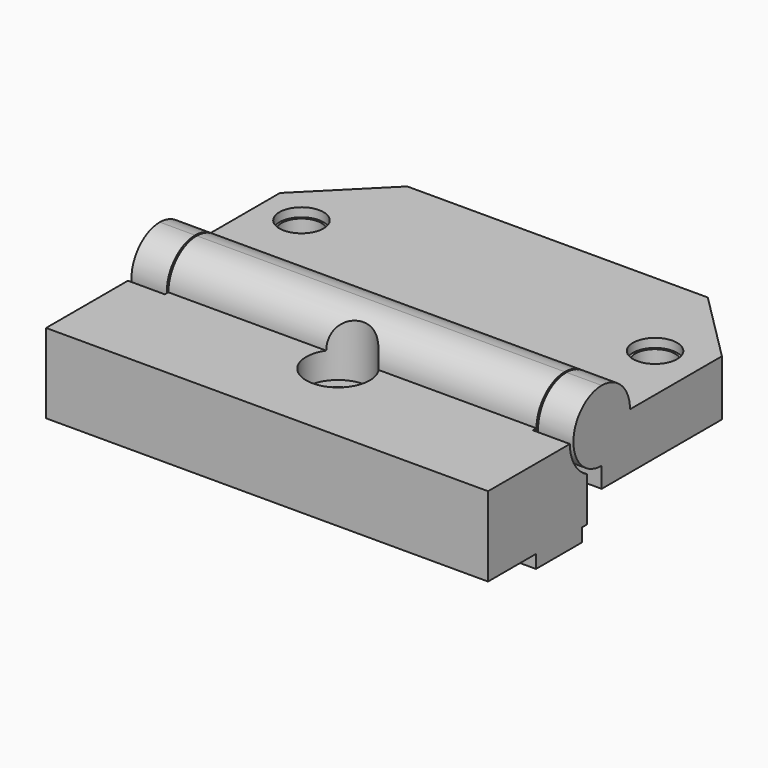
from build123d import *

# Parameters (mm, degrees)
F4_W           = 41.6464466094
F4_H           = 8
F6_W           = 4
F6_H           = 8
F7_DEPTH       = 25
F8_DEPTH       = 42
F10_DEPTH      = 46.001
F14_DEPTH      = 4
F14_DEPTH_BACK = 46
F15_DEPTH      = 41.6464466094
F16_DEPTH      = 4.1767766953
F16_DEPTH_BACK = 45.8232233047
F17_W          = 49.9999999998
F17_H          = 8.9284215122
F17_R          = 2.25
F18_DEPTH      = 25
F20_DEPTH      = 5
F21_R          = 2.25
F22_DEPTH      = 25
F23_R          = 3.6
F24_DEPTH      = 3
F24_DEPTH_BACK = 25
F25_W          = 50.0000000003
F25_H          = 6.5
F25_R          = 2.25
F26_DEPTH      = 1.5
F27_R          = 2.25
F28_DEPTH      = 25
F30_DEPTH      = 2.3
F31_R          = 2.25
F32_DEPTH      = 25
F33_SIZE       = 8
F34_R          = 2
F35_DEPTH      = 4.2
F36_R          = 2.5
F37_DEPTH      = 1


with BuildPart() as f1:
    # F0 (on Top) → F1 (revolve)
    with BuildSketch(Plane.XY):
        Polygon((-25, 0), (-17, 0), (-21, 4), (-25, 4), align=None)
    revolve(axis=Axis((-8.4116116524, 0, 0), (-1, 0, 0)))

    # F6 (on offset) → F7, piece 2 (join, through all)
    with BuildSketch(Plane.XZ.offset(-25)):
        with Locations((-23, 0)):
            Rectangle(F6_W, F6_H)
    extrude(amount=F7_DEPTH)


with BuildPart() as f1b:
    # F0 (on Top) → F1, piece 2 (revolve)
    with BuildSketch(Plane.XY):
        Polygon((-16.8232233047, 0), (0, 0), (0, 4), (-20.8232233047, 4), align=None)
        Polygon((0, 4), (0, 0), (16.8232233047, 0), (20.8232233047, 4), align=None)
    revolve(axis=Axis((-8.4116116524, 0, 0), (-1, 0, 0)))

    # F4 (on offset) → F5 (join, up to the next surface of F1b)
    with BuildSketch(Plane.XZ.offset(25)):
        Rectangle(F4_W, F4_H)
    extrude(until=Until.NEXT, dir=(0, 1, 0))

    # F13 (on face) → F15 (cut, through all)
    with BuildSketch(Plane.YZ.offset(20.8232233047)):
        with BuildLine():
            Line((-25, 4), (-25, 0))
            Line((-25, 0), (-4.5, 0))
            Line((-4.5, 0), (-4, 0))
            ThreePointArc((-4, 0), (-2.8284271247, 2.8284271247), (0, 4))
            Line((0, 4), (-25, 4))
        make_face()
    extrude(amount=-F15_DEPTH, mode=Mode.SUBTRACT)

    # F13 (on face) → F16 (join, two sides)
    with BuildSketch(Plane.YZ.offset(20.8232233047)) as f16_sk:
        with BuildLine():
            Line((-4.5, 0), (-25, 0))
            Line((-25, 0), (-25, -4))
            Line((-25, -4), (-2.0615528128, -4))
            ThreePointArc((-2.0615528128, -4), (-3.8423292192, -2.3423292192), (-4.5, 0))
        make_face()
    extrude(amount=F16_DEPTH)
    extrude(f16_sk.sketch, amount=-F16_DEPTH_BACK)

    # F17 (on face) → F18 (cut)
    with BuildSketch(Plane.XY):
        with Locations((-1e-10, -20.5357892439)):
            Rectangle(F17_W, F17_H)
        with Locations((-1e-10, -6.0417063069)):
            Circle(F17_R)
    extrude(amount=-F18_DEPTH, mode=Mode.SUBTRACT)

    # F19 (on face) → F20 (join)
    with BuildSketch(Plane(origin=(0, 0, -4), x_dir=(1, 0, 0), z_dir=(0, 0, -1))):
        Polygon((25, 16.0715784878), (-25, 16.0715784878), (-25, 2.0615528128), (-20.8232233047, 2.0615528128), (-20.8232233047, 0), (20.8232233047, 0), (20.8232233047, 2.0615528128), (25, 2.0615528128), align=None)
    extrude(amount=F20_DEPTH)

    # F21 (on face) → F22 (cut)
    with BuildSketch(Plane.XY):
        with Locations((-1e-10, -6.0417063069)):
            Circle(F21_R)
    extrude(amount=-F22_DEPTH, mode=Mode.SUBTRACT)

    # F23 (on face) → F24 (cut, two sides)
    with BuildSketch(Plane.XY) as f24_sk:
        with Locations((-1e-10, -6.0417063069)):
            Circle(F23_R)
    extrude(amount=-F24_DEPTH, mode=Mode.SUBTRACT)
    extrude(f24_sk.sketch, amount=F24_DEPTH_BACK, mode=Mode.SUBTRACT)

    # F25 (on face) → F26 (join)
    with BuildSketch(Plane(origin=(0, 0, -9), x_dir=(1, 0, 0), z_dir=(0, 0, -1))):
        with Locations((-1e-10, 6.0417063069)):
            Rectangle(F25_W, F25_H)
        with Locations((-1e-10, 6.0417063069)):
            Circle(F25_R, mode=Mode.SUBTRACT)
    extrude(amount=F26_DEPTH)


with BuildPart() as f1c:
    # F0 (on Top) → F1, piece 3 (revolve)
    with BuildSketch(Plane.XY):
        Polygon((25, 4), (21, 4), (17, 0), (25, 0), align=None)
    revolve(axis=Axis((-8.4116116524, 0, 0), (-1, 0, 0)))

    # F6 (on offset) → F7 (join, through all)
    with BuildSketch(Plane.XZ.offset(-25)):
        with Locations((23, 0)):
            Rectangle(F6_W, F6_H)
    extrude(amount=F7_DEPTH)


with BuildPart() as f8:
    # F8 (new, through all): a face of the model
    f8_faces = [f1.part.faces().sort_by_distance(p)[0] for p in [
        (-21, 14.0525639311, 0),
    ]]
    extrude(f8_faces, amount=F8_DEPTH)

    # F9 (on face) → F10 (cut, through all)
    with BuildSketch(Plane(origin=(-21, 0, 0), x_dir=(0, -1, 0), z_dir=(-1, 0, 0))):
        with BuildLine():
            Line((-8.5, -4), (0, -4))
            ThreePointArc((0, -4), (-4, 0), (0, 4))
            Line((0, 4), (-8.5, 4))
            ThreePointArc((-8.5, 4), (-4.5, 0), (-8.5, -4))
        make_face()
    extrude(amount=-F10_DEPTH, mode=Mode.SUBTRACT)


with BuildPart() as f1c_1:
    add(f1c.part)

    # F12: union F8, F1
    add(f8.part)
    add(f1.part)

    # F11 (on face) → F14 (cut, two sides)
    with BuildSketch(Plane.YZ.offset(-21)) as f14_sk:
        with BuildLine():
            Line((4, 0), (25, 0))
            Line((25, 0), (25, 4))
            Line((25, 4), (0, 4))
            ThreePointArc((0, 4), (2.8284271247, 2.8284271247), (4, 0))
        make_face()
    extrude(amount=-F14_DEPTH, mode=Mode.SUBTRACT)
    extrude(f14_sk.sketch, amount=F14_DEPTH_BACK, mode=Mode.SUBTRACT)

    # F27 (on face) → F28 (cut)
    with BuildSketch(Plane(origin=(0, 0, -4), x_dir=(1, 0, 0), z_dir=(0, 0, -1))):
        with Locations((-20.2462286502, -14.1022969037)):
            Circle(F27_R)
        with Locations((19.7537713498, -14.1022969037)):
            Circle(F27_R)
    extrude(amount=-F28_DEPTH, mode=Mode.SUBTRACT)

    # F29 (on face) → F30 (join)
    with BuildSketch(Plane(origin=(0, 0, -4), x_dir=(1, 0, 0), z_dir=(0, 0, -1))):
        Polygon((-25, -8.5), (-25, -25), (25, -25), (25, -8.5), (25, 0), (21, 0), (21, -8.5), (-21, -8.5), (-21, 0), (-25, 0), align=None)
    extrude(amount=F30_DEPTH)

    # F31 (on face) → F32 (cut)
    with BuildSketch(Plane.XY):
        with Locations((-20.2462286502, 14.1022969037)):
            Circle(F31_R)
        with Locations((19.7537713498, 14.1022969037)):
            Circle(F31_R)
    extrude(amount=-F32_DEPTH, mode=Mode.SUBTRACT)

    # F33
    f33_edges = [f1c_1.edges().sort_by_distance(p)[0] for p in [
        (-25, 25, -2),
        (-25, 25, -5.15),
        (25, 25, -2),
        (25, 25, -5.15),
    ]]
    chamfer(f33_edges, length=F33_SIZE)

    # F34 (on face) → F35 (join)
    with BuildSketch(Plane(origin=(0, 0, -6.3), x_dir=(1, 0, 0), z_dir=(0, 0, -1))):
        with Locations((0, -20.9749843925)):
            Circle(F34_R)
    extrude(amount=F35_DEPTH)

    # F36 (on face) → F37 (cut)
    with BuildSketch(Plane.XY):
        with Locations((-20.2462286502, 14.1022969037)):
            Circle(F36_R)
        with Locations((19.7537713498, 14.1022969037)):
            Circle(F36_R)
    extrude(amount=-F37_DEPTH, mode=Mode.SUBTRACT)


solid = Compound([f1b.part, f1c_1.part])
